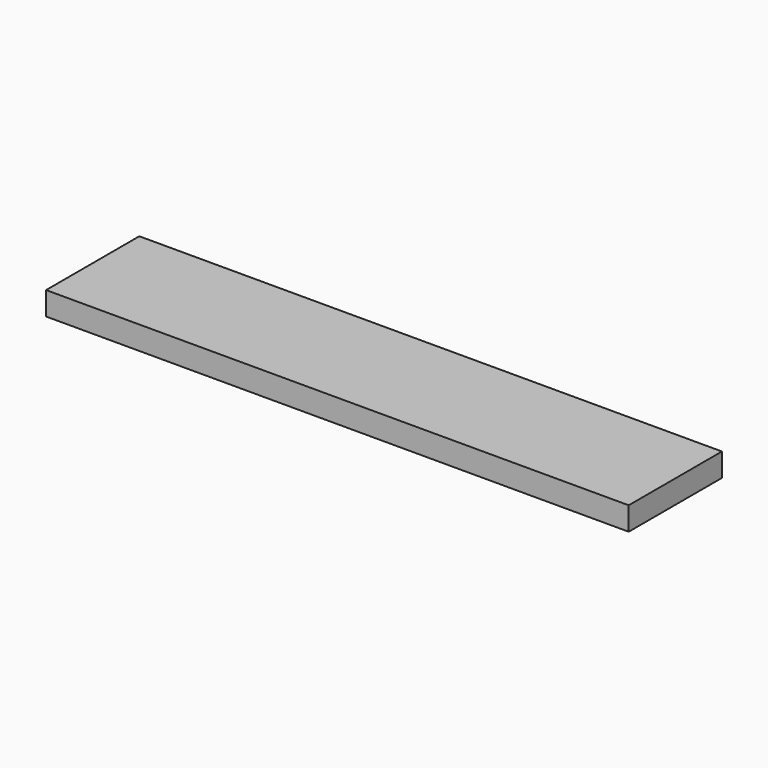
from build123d import *

# Parameters (mm, degrees)
F0_W         = 50
F0_H         = 10
F1_DEPTH     = 2
F2_TEXT_SIZE = 10.9971319703
F3_DEPTH     = 1


# Not quite as in the source:
# - Text() gives the source's letters only with a copy of the font that has no kerning and outlines rounded to 1/6400 em; it was checked with that copy


with BuildPart() as f1:
    # F0 (on Top) → F1 (new body)
    with BuildSketch(Plane.XY):
        Rectangle(F0_W, F0_H)
    extrude(amount=F1_DEPTH)

    # F2 (on face) → F3 (cut)
    with BuildSketch(Plane(origin=(0, 0, 0), x_dir=(1, 0, 0), z_dir=(0, 0, -1))):
        with Locations((-12.7223070481, -3.9589675093)):
            Text('TEST', F2_TEXT_SIZE, font='Open Sans', font_style=FontStyle.BOLD, text_align=(TextAlign.LEFT, TextAlign.BOTTOM))
    extrude(amount=-F3_DEPTH, mode=Mode.SUBTRACT)


solid = f1.part
